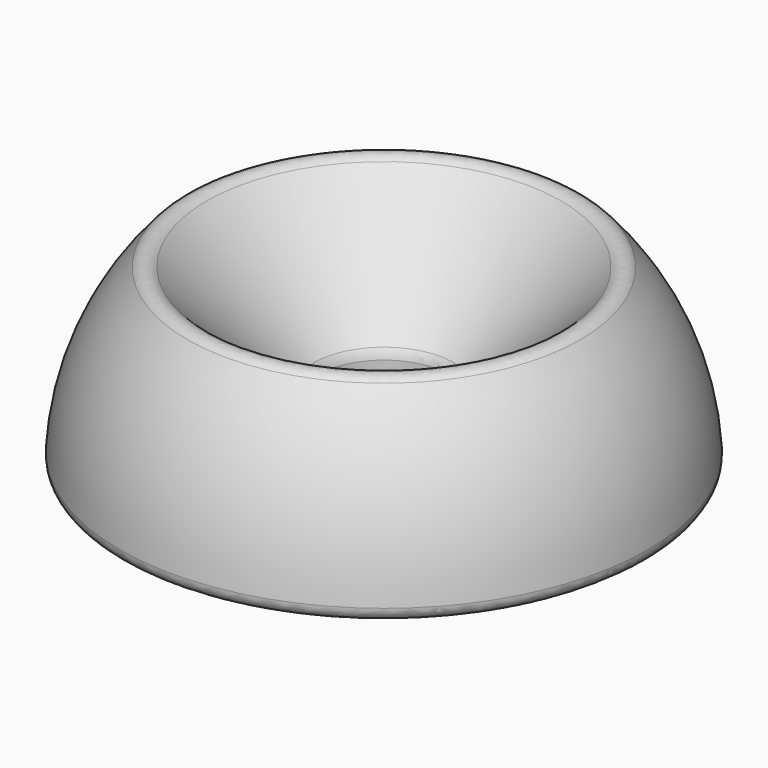
from build123d import *

# Parameters (mm, degrees)
F2_R = 1


with BuildPart() as f1:
    # F0 (on Front) → F1 (revolve)
    with BuildSketch(Plane.XZ):
        with BuildLine():
            ThreePointArc((20, 0), (18.4775906502, 7.6536686473), (14.1421356237, 14.1421356237))
            Line((14.1421356237, 14.1421356237), (5, 5))
            Line((5, 5), (5, 0))
            Line((5, 0), (20, 0))
        make_face()
    revolve(axis=Axis((0, 0, 1.4953076416), (0, 0, -1)))

    # F2
    f2_edges = [f1.edges().sort_by_distance(p)[0] for p in [
        (-5, 0, 5),
        (-14.142136, 0, 14.142136),
        (-20, 0, 0),
    ]]
    fillet(f2_edges, radius=F2_R)


solid = f1.part
